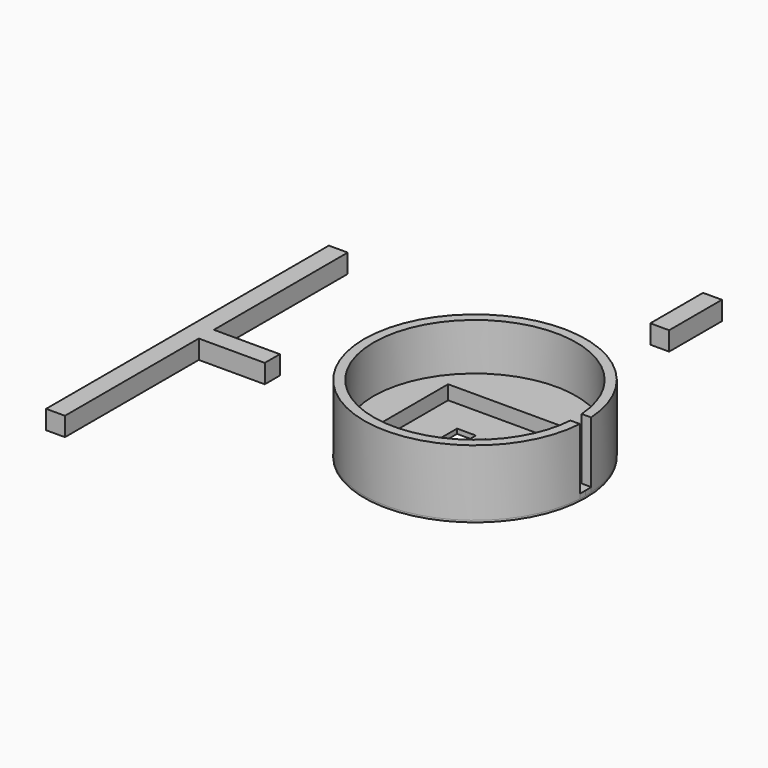
from build123d import *
from build123d import SkipClean  # not in build123d's __all__

# Parameters (mm, degrees)
F2_DEPTH = 7
F3_DEPTH = 2
F0_W     = 14.5
F0_H     = 11
F0_W_2   = 2
F0_H_2   = 4
F4_DEPTH = 0.5
F5_DEPTH = 0.5
F1_R     = 11.75
F1_R_2   = 11.25
F6_DEPTH = 0.2
F7_W     = 7
F7_H     = 2
F8_DEPTH = 2
F7_W_2   = 2
F7_H_2   = 7


with BuildPart() as f2:
    # F0 (on Top) → F2 (new body)
    with BuildSketch(Plane.XY):
        with BuildLine():
            ThreePointArc((9.236476601, 5.5), (10.258841959, 3.2122673707), (10.7238052948, 0.75))
            Line((10.7238052948, 0.75), (11.7260393996, 0.75))
            ThreePointArc((11.7260393996, 0.75), (-11.75, 0), (11.7260393996, -0.75))
            Line((11.7260393996, -0.75), (10.7238052948, -0.75))
            ThreePointArc((10.7238052948, -0.75), (10.258841959, -3.2122673707), (9.236476601, -5.5))
            ThreePointArc((9.236476601, -5.5), (-10.75, 0), (9.236476601, 5.5))
        make_face()
    extrude(amount=F2_DEPTH)

    # F0 (on Top) → F3 (join)
    with BuildSketch(Plane.XY):
        with BuildLine():
            Line((7.25, 5.5), (9.236476601, 5.5))
            ThreePointArc((9.236476601, 5.5), (-10.75, 0), (9.236476601, -5.5))
            Line((9.236476601, -5.5), (7.25, -5.5))
            Line((7.25, -5.5), (-7.25, -5.5))
            Line((-7.25, -5.5), (-7.25, 5.5))
            Line((-7.25, 5.5), (7.25, 5.5))
        make_face()
    extrude(amount=F3_DEPTH)

    # F0 (on Top) → F4 (join)
    with BuildSketch(Plane.XY):
        Rectangle(F0_W, F0_H)
        with Locations((-2.5, 0)):
            Rectangle(F0_W_2, F0_H_2, mode=Mode.SUBTRACT)
        with Locations((0.5, 0)):
            Rectangle(F0_W_2, F0_H_2, mode=Mode.SUBTRACT)
    extrude(amount=F4_DEPTH)

    # F0 (on Top) → F5 (join)
    with BuildSketch(Plane.XY):
        with BuildLine():
            ThreePointArc((10.7238052948, -0.75), (10.7434493278, -0.3752286512), (10.75, 0))
            ThreePointArc((10.75, 0), (10.7434493278, 0.3752286512), (10.7238052948, 0.75))
            ThreePointArc((10.7238052948, 0.75), (10.258841959, 3.2122673707), (9.236476601, 5.5))
            Line((9.236476601, 5.5), (7.25, 5.5))
            Line((7.25, 5.5), (7.25, -5.5))
            Line((7.25, -5.5), (9.236476601, -5.5))
            ThreePointArc((9.236476601, -5.5), (10.258841959, -3.2122673707), (10.7238052948, -0.75))
        make_face()
        with BuildLine():
            ThreePointArc((10.7238052948, 0.75), (10.7434493278, 0.3752286512), (10.75, 0))
            ThreePointArc((10.75, 0), (10.7434493278, -0.3752286512), (10.7238052948, -0.75))
            Line((10.7238052948, -0.75), (11.7260393996, -0.75))
            ThreePointArc((11.7260393996, -0.75), (11.7440083222, -0.3751913213), (11.75, 0))
            ThreePointArc((11.75, 0), (11.7440083222, 0.3751913213), (11.7260393996, 0.75))
            Line((11.7260393996, 0.75), (10.7238052948, 0.75))
        make_face()
    extrude(amount=F5_DEPTH)

    # F1 (on face) → F6 (join)
    with BuildSketch(Plane.XY):
        Circle(F1_R)
        Circle(F1_R_2, mode=Mode.SUBTRACT)
        with BuildLine():
            ThreePointArc((6.9971422738, -5.5), (8.4108431871, -2.9099341713), (8.9, 0))
            ThreePointArc((8.9, 0), (8.4108431871, 2.9099341713), (6.9971422738, 5.5))
            Line((6.9971422738, 5.5), (6.3490156717, 5.5))
            ThreePointArc((6.3490156717, 5.5), (7.8705695995, 2.9349845278), (8.4, 0))
            ThreePointArc((8.4, 0), (7.8705695995, -2.9349845278), (6.3490156717, -5.5))
            Line((6.3490156717, -5.5), (6.9971422738, -5.5))
        make_face()
        with BuildLine():
            ThreePointArc((-6.9971422738, -5.5), (0, -8.9), (6.9971422738, -5.5))
            Line((6.9971422738, -5.5), (6.3490156717, -5.5))
            ThreePointArc((6.3490156717, -5.5), (0, -8.4), (-6.3490156717, -5.5))
            Line((-6.3490156717, -5.5), (-6.9971422738, -5.5))
        make_face()
        with BuildLine():
            ThreePointArc((-7.25, -5.1621216568), (-7.1255740952, -5.3325597806), (-6.9971422738, -5.5))
            Line((-6.9971422738, -5.5), (-6.3490156717, -5.5))
            ThreePointArc((-6.3490156717, -5.5), (-6.8285232792, -4.8919597121), (-7.25, -4.2423460491))
            Line((-7.25, -4.2423460491), (-7.25, -5.1621216568))
        make_face()
        with BuildLine():
            Line((-7.25, 4.2423460491), (-7.25, 5.1621216568))
            ThreePointArc((-7.25, 5.1621216568), (-8.9, 0), (-7.25, -5.1621216568))
            Line((-7.25, -5.1621216568), (-7.25, -4.2423460491))
            ThreePointArc((-7.25, -4.2423460491), (-8.4, 0), (-7.25, 4.2423460491))
        make_face()
        with BuildLine():
            Line((6.3490156717, 5.5), (6.9971422738, 5.5))
            ThreePointArc((6.9971422738, 5.5), (0, 8.9), (-6.9971422738, 5.5))
            Line((-6.9971422738, 5.5), (-6.3490156717, 5.5))
            ThreePointArc((-6.3490156717, 5.5), (0, 8.4), (6.3490156717, 5.5))
        make_face()
        with BuildLine():
            Line((-6.3490156717, 5.5), (-6.9971422738, 5.5))
            ThreePointArc((-6.9971422738, 5.5), (-7.1255740952, 5.3325597806), (-7.25, 5.1621216568))
            Line((-7.25, 5.1621216568), (-7.25, 4.2423460491))
            ThreePointArc((-7.25, 4.2423460491), (-6.8285232792, 4.8919597121), (-6.3490156717, 5.5))
        make_face()
    with SkipClean():  # cleaning this boolean's faces spoils the solid; the shape is the same uncleaned
        extrude(amount=-F6_DEPTH)


with BuildPart() as f8:
    # F7 (on Top) → F8 (new body)
    with BuildSketch(Plane.XY):
        Polygon((-28.5, 18.75), (-30.5, 18.75), (-30.5, -18.75), (-28.5, -18.75), (-28.5, -1), (-28.5, 1), align=None)
        with Locations((-25, 0)):
            Rectangle(F7_W, F7_H)
    extrude(amount=F8_DEPTH)


with BuildPart() as f8b:
    # F7 (on Top) → F8, piece 2 (new body)
    with BuildSketch(Plane.XY):
        with Locations((0, 28)):
            Rectangle(F7_W_2, F7_H_2)
    extrude(amount=F8_DEPTH)


solid = Compound([f2.part, f8.part, f8b.part])
